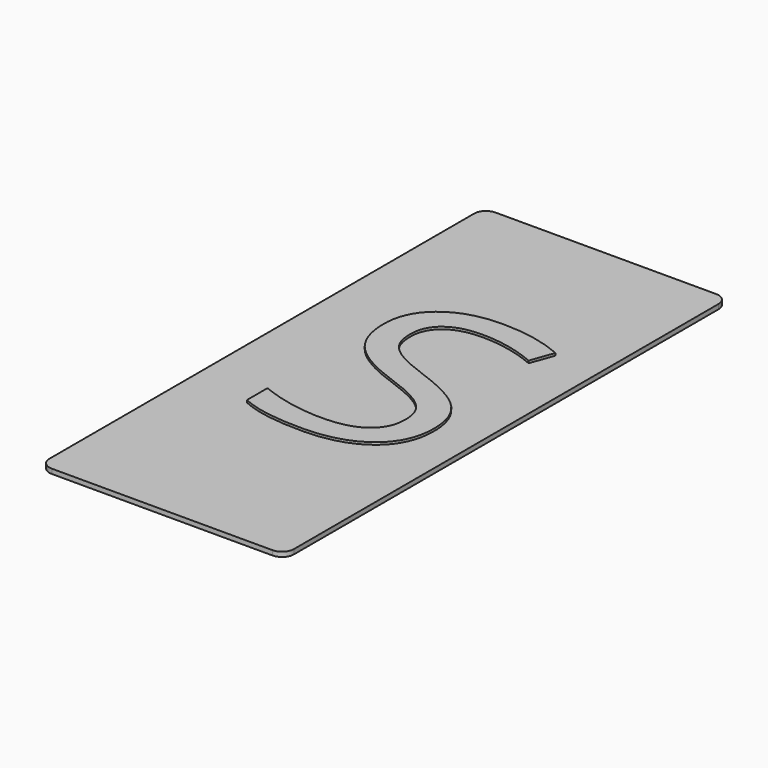
from build123d import *

# Parameters (mm, degrees)
F0_W         = 104.14
F0_H         = 236.22
F1_DEPTH     = 2
F2_TEXT_SIZE = 136.7496895707
F3_DEPTH     = 1
F4_R         = 5.08


# Not quite as in the source:
# - Text() gives the source's letters only with a copy of the font that has no kerning and outlines rounded to 1/6400 em; it was checked with that copy


with BuildPart() as f1:
    # F0 (on Top) → F1 (new body)
    with BuildSketch(Plane.XY):
        with Locations((1.2983363122, 87.63)):
            Rectangle(F0_W, F0_H)
    extrude(amount=F1_DEPTH)

    # F2 (on face) → F3 (join)
    with BuildSketch(Plane.XY.offset(2)):
        with Locations((-31.7703627516, 44.0382398665)):
            Text('S', F2_TEXT_SIZE, font='Open Sans', text_align=(TextAlign.LEFT, TextAlign.BOTTOM))
    extrude(amount=F3_DEPTH)

    # F4
    f4_edges = [f1.edges().sort_by_distance(p)[0] for p in [
        (-50.771664, 205.74, 1),
        (53.368336, 205.74, 1),
        (-50.771664, -30.48, 1),
        (53.368336, -30.48, 1),
    ]]
    fillet(f4_edges, radius=F4_R)


solid = f1.part
